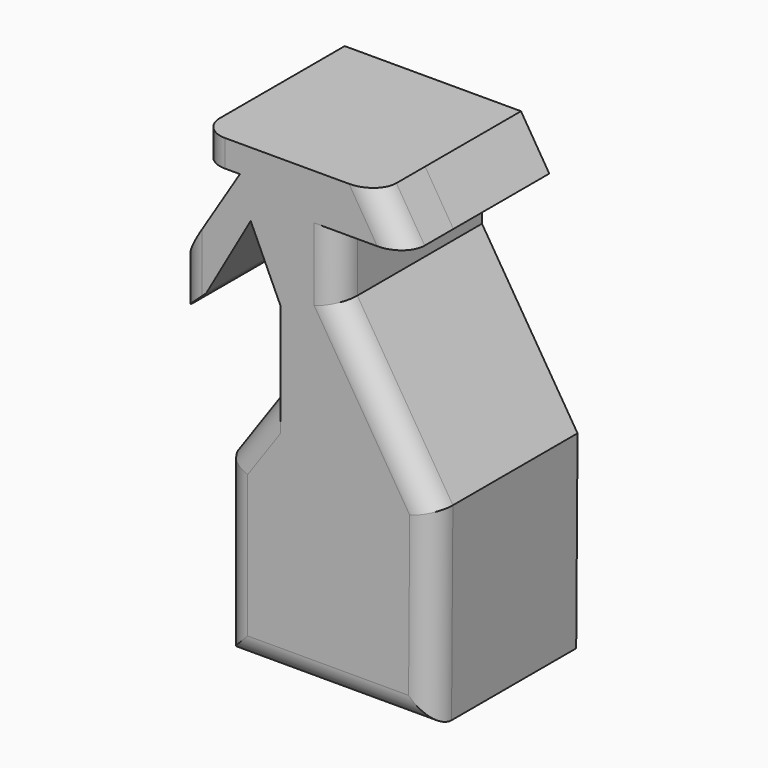
from build123d import *

# Parameters (mm, degrees)
F1_DEPTH = 12.7
F2_DEPTH = 25.4
F3_R     = 5.08


with BuildPart() as f1:
    # F0 (on Front) → F1 (new body)
    with BuildSketch(Plane.XZ):
        Polygon((-29.3797869235, -7.2736367583), (-29.3797869235, -44.0696775913), (14.8325152695, -44.0696775913), (15.1177551597, -3.8507485297), (-5.1343315281, 28.666684404), (-5.1343315281, 42.6434762776), (9.1277007014, 42.6434762776), (3.1376483385, 52.341658622), (-34.2288762331, 52.341658622), (-34.2288762331, 46.6368459165), (-25.9568989277, 46.6368459165), (-39.0779674053, 25.529038161), (-39.0779674053, 16.6865773499), (-33.0879166722, 22.1061483026), (-23.674974218, 38.6501066387), (-17.3996798694, 24.958556518), (-17.3996798694, 9.8408022895), align=None)
    extrude(amount=F1_DEPTH)

    # F0 (on Front) + F1_face (on face) + F1_face1 (on face) → F2 (join)
    with BuildSketch(Plane.XZ):
        Polygon((-29.3797869235, -7.2736367583), (-29.3797869235, -44.0696775913), (14.8325152695, -44.0696775913), (15.1177551597, -3.8507485297), (-5.1343315281, 28.666684404), (-5.1343315281, 42.6434762776), (9.1277007014, 42.6434762776), (3.1376483385, 52.341658622), (-34.2288762331, 52.341658622), (-34.2288762331, 46.6368459165), (-25.9568989277, 46.6368459165), (-39.0779674053, 25.529038161), (-39.0779674053, 16.6865773499), (-33.0879166722, 22.1061483026), (-23.674974218, 38.6501066387), (-17.3996798694, 24.958556518), (-17.3996798694, 9.8408022895), align=None)
    with BuildSketch(Plane(origin=(-9.327897656, -12.7, -1.3317405801), x_dir=(1, 0, 0), z_dir=(0, -1, 0))):
        Polygon((18.4555983573, 43.9752168577), (12.4655459944, 53.6733992022), (-24.9009785771, 53.6733992022), (-24.9009785771, 47.9685864966), (-16.6290012717, 47.9685864966), (-29.7500697493, 26.8607787412), (-29.7500697493, 18.01831793), (-23.7600190162, 23.4378888827), (-14.347076562, 39.9818472188), (-8.0717822134, 26.2902970981), (-8.0717822134, 11.1725428697), (-20.0518892675, -5.9418961782), (-20.0518892675, -42.7379370112), (24.1604129255, -42.7379370112), (24.4456528157, -2.5190079495), (4.1935661279, 29.9984249842), (4.1935661279, 43.9752168577), align=None)
    with BuildSketch(Plane(origin=(-9.327897656, 0, -1.3317405801), x_dir=(1, 0, 0), z_dir=(0, 1, 0))):
        Polygon((12.4655459944, -53.6733992022), (18.4555983573, -43.9752168577), (4.1935661279, -43.9752168577), (4.1935661279, -29.9984249842), (24.4456528157, 2.5190079495), (24.1604129255, 42.7379370112), (-20.0518892675, 42.7379370112), (-20.0518892675, 5.9418961782), (-8.0717822134, -11.1725428697), (-8.0717822134, -26.2902970981), (-14.347076562, -39.9818472188), (-23.7600190162, -23.4378888827), (-29.7500697493, -18.01831793), (-29.7500697493, -26.8607787412), (-16.6290012717, -47.9685864966), (-24.9009785771, -47.9685864966), (-24.9009785771, -53.6733992022), align=None)
    extrude(amount=F2_DEPTH, dir=(0, -1, 0))

    # F3
    f3_edges = [f1.edges().sort_by_distance(p)[0] for p in [
        (-39.077967, -38.1, 21.107808),
        (-36.082942, 0, 19.396363),
        (6.132675, -38.1, 47.492567),
        (4.991712, -38.1, 12.407968),
        (-5.134332, -38.1, 35.65508),
        (14.975135, -38.1, -23.960213),
        (-34.228876, -38.1, 49.489252),
        (-23.389733, -38.1, 1.283583),
        (-29.379787, -38.1, -25.671657),
        (-7.273636, -38.1, -44.069678),
    ]]
    fillet(f3_edges, radius=F3_R)


solid = f1.part
